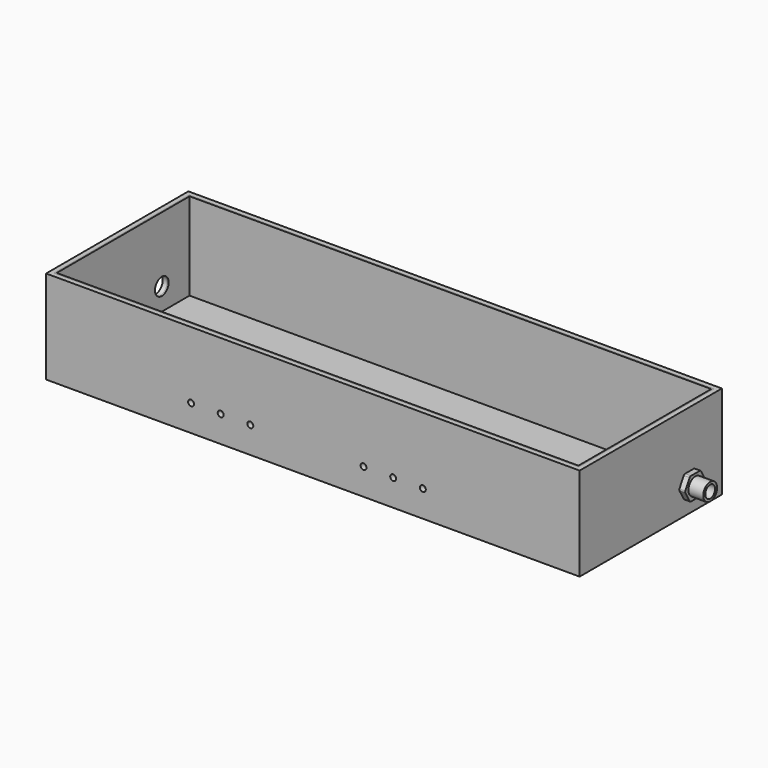
from build123d import *

# Parameters (mm, degrees)
F0_W      = 900
F0_H      = 300
F1_DEPTH  = 7.5
F2_W      = 900
F2_H      = 300
F2_W_2    = 885
F2_H_2    = 285
F3_DEPTH  = 150
F4_DEPTH  = 2.5
F5_W      = 885
F5_H      = 285
F5_W_2    = 880
F5_H_2    = 280
F6_DEPTH  = 147.5
F7_R      = 5
F8_DEPTH  = 25
F9_R      = 14.39
F10_DEPTH = 500
F11_R     = 14.39
F12_DEPTH = 25
F13_R     = 14.39
F13_R_2   = 10.39
F14_DEPTH = 10
F15_R     = 10.39
F16_DEPTH = 10
F17_R     = 14.6154428136
F17_R_2   = 10.39
F18_DEPTH = 25
F19_R     = 11.2359155228
F19_R_2   = 8.5030368104
F20_DEPTH = 50
F21_R     = 11.2359155228
F22_DEPTH = 10


with BuildPart() as f1:
    # F0 (on Top) → F1 (new body)
    with BuildSketch(Plane.XY):
        Rectangle(F0_W, F0_H)
    extrude(amount=F1_DEPTH)

    # F2 (on face) → F3 (join)
    with BuildSketch(Plane.XY.offset(7.5)):
        Rectangle(F2_W, F2_H)
        Rectangle(F2_W_2, F2_H_2, mode=Mode.SUBTRACT)
    extrude(amount=F3_DEPTH)


with BuildPart() as f4:
    # F4 (new): a face of the model
    f4_faces = [f1.part.faces().sort_by_distance(p)[0] for p in [
        (0, 0, 7.5),
    ]]
    extrude(f4_faces, amount=F4_DEPTH)

    # F5 (on face) → F6 (join)
    with BuildSketch(Plane.XY.offset(10)):
        Rectangle(F5_W, F5_H)
        Rectangle(F5_W_2, F5_H_2, mode=Mode.SUBTRACT)
    extrude(amount=F6_DEPTH)


with BuildPart() as f8_tool:
    # F7 (on face) → F8 (new body)
    with BuildSketch(Plane.XZ.offset(150)):
        with Locations((85.5, 44.781)):
            Circle(F7_R)
        with Locations((135.5, 44.781)):
            Circle(F7_R)
        with Locations((-105.5, 44.78)):
            Circle(F7_R)
        with Locations((-155.5, 44.78)):
            Circle(F7_R)
        with Locations((185.5, 44.781)):
            Circle(F7_R)
        with Locations((-205.5, 44.78)):
            Circle(F7_R)
    extrude(amount=-F8_DEPTH)


with BuildPart() as f1_1:
    add(f1.part)

    # F8: cut by f8_tool
    add(f8_tool.part, mode=Mode.SUBTRACT)


with BuildPart() as f4_1:
    add(f4.part)

    # F8: cut by f8_tool
    add(f8_tool.part, mode=Mode.SUBTRACT)


with BuildPart() as f10_tool:
    # F9 (on face) → F10 (new body)
    with BuildSketch(Plane(origin=(-450, 0, 0), x_dir=(0, -1, 0), z_dir=(-1, 0, 0))):
        with Locations((-81.5, 47.5)):
            Circle(F9_R)
    extrude(amount=-F10_DEPTH)


with BuildPart() as f1_2:
    add(f1_1.part)

    # F10: cut by f10_tool
    add(f10_tool.part, mode=Mode.SUBTRACT)


with BuildPart() as f4_2:
    add(f4_1.part)

    # F10: cut by f10_tool
    add(f10_tool.part, mode=Mode.SUBTRACT)


with BuildPart() as f12_tool:
    # F11 (on face) → F12 (new body)
    with BuildSketch(Plane.YZ.offset(450)):
        with Locations((81.5, 43.5)):
            Circle(F11_R)
    extrude(amount=-F12_DEPTH)


with BuildPart() as f1_3:
    add(f1_2.part)

    # F12: cut by f12_tool
    add(f12_tool.part, mode=Mode.SUBTRACT)


with BuildPart() as f4_3:
    add(f4_2.part)

    # F12: cut by f12_tool
    add(f12_tool.part, mode=Mode.SUBTRACT)


with BuildPart() as f14:
    # F13 (on face) → F14 (new body)
    with BuildSketch(Plane.YZ.offset(450)):
        with Locations((81.5, 43.5)):
            Circle(F13_R)
        with Locations((81.5, 43.5)):
            Circle(F13_R_2, mode=Mode.SUBTRACT)
    extrude(amount=-F14_DEPTH)

    # F15 (on face) → F16 (join)
    with BuildSketch(Plane.YZ.offset(450)):
        with BuildLine():
            Line((90.7447234463, 62.5123307109), (72.2552765537, 62.5123307109))
            ThreePointArc((72.2552765537, 62.5123307109), (70.7552765537, 62.1104069222), (69.6572003424, 61.0123307109))
            Line((69.6572003424, 61.0123307109), (60.4124768961, 45))
            ThreePointArc((60.4124768961, 45), (60.0105531074, 43.5), (60.4124768961, 42))
            Line((60.4124768961, 42), (69.6572003424, 25.9876692891))
            ThreePointArc((69.6572003424, 25.9876692891), (70.7552765537, 24.8895930778), (72.2552765537, 24.4876692891))
            Line((72.2552765537, 24.4876692891), (90.7447234463, 24.4876692891))
            ThreePointArc((90.7447234463, 24.4876692891), (92.2447234463, 24.8895930778), (93.3427996576, 25.9876692891))
            Line((93.3427996576, 25.9876692891), (102.5875231039, 42))
            ThreePointArc((102.5875231039, 42), (102.9894468926, 43.5), (102.5875231039, 45))
            Line((102.5875231039, 45), (93.3427996576, 61.0123307109))
            ThreePointArc((93.3427996576, 61.0123307109), (92.2447234463, 62.1104069222), (90.7447234463, 62.5123307109))
        make_face()
        with Locations((81.5, 43.5)):
            Circle(F15_R, mode=Mode.SUBTRACT)
    extrude(amount=F16_DEPTH)

    # F17 (on face) → F18 (join)
    with BuildSketch(Plane.YZ.offset(460)):
        with Locations((81.5, 43.5)):
            Circle(F17_R)
        with Locations((81.5, 43.5)):
            Circle(F17_R_2, mode=Mode.SUBTRACT)
    extrude(amount=F18_DEPTH)

    # F19 (on face) → F20 (join)
    with BuildSketch(Plane(origin=(440, 0, 0), x_dir=(0, -1, 0), z_dir=(-1, 0, 0))):
        with Locations((-81.5, 43.5)):
            Circle(F19_R)
        with Locations((-81.5, 43.5)):
            Circle(F19_R_2, mode=Mode.SUBTRACT)
    extrude(amount=F20_DEPTH)

    # F21 (on face) → F22 (join)
    with BuildSketch(Plane(origin=(440, 0, 0), x_dir=(0, -1, 0), z_dir=(-1, 0, 0))):
        with BuildLine():
            Line((-72.2552765537, 62.5123307109), (-90.7447234463, 62.5123307109))
            ThreePointArc((-90.7447234463, 62.5123307109), (-92.2447234463, 62.1104069222), (-93.3427996576, 61.0123307109))
            Line((-93.3427996576, 61.0123307109), (-102.5875231039, 45))
            ThreePointArc((-102.5875231039, 45), (-102.9894468926, 43.5), (-102.5875231039, 42))
            Line((-102.5875231039, 42), (-93.3427996576, 25.9876692891))
            ThreePointArc((-93.3427996576, 25.9876692891), (-92.2447234463, 24.8895930778), (-90.7447234463, 24.4876692891))
            Line((-90.7447234463, 24.4876692891), (-72.2552765537, 24.4876692891))
            ThreePointArc((-72.2552765537, 24.4876692891), (-70.7552765537, 24.8895930778), (-69.6572003424, 25.9876692891))
            Line((-69.6572003424, 25.9876692891), (-60.4124768961, 42))
            ThreePointArc((-60.4124768961, 42), (-60.0105531074, 43.5), (-60.4124768961, 45))
            Line((-60.4124768961, 45), (-69.6572003424, 61.0123307109))
            ThreePointArc((-69.6572003424, 61.0123307109), (-70.7552765537, 62.1104069222), (-72.2552765537, 62.5123307109))
        make_face()
        with Locations((-81.5, 43.5)):
            Circle(F21_R, mode=Mode.SUBTRACT)
    extrude(amount=F22_DEPTH)


solid = Compound([f1_3.part, f4_3.part, f14.part])
